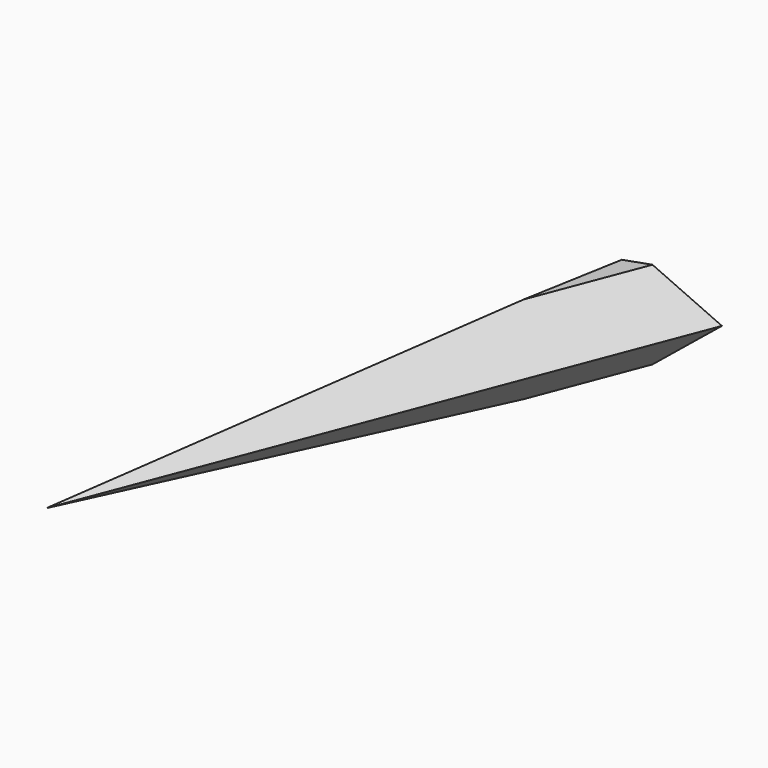
from build123d import *

# Parameters (mm, degrees)
F1_DEPTH = 10
F2_SIZE  = 4.99999


# Not quite as in the source:
# - a fillet or chamfer is up to 0.001 mm smaller than in the source, because OpenCascade refuses the exact size


with BuildPart() as f1:
    # F0 (on Top) → F1 (new body)
    with BuildSketch(Plane.XY):
        Polygon((-26.4395750973, 41.8424181081), (-40.7729081464, 36.8424181081), (-51.4395743695, -23.1575818919), align=None)
    extrude(amount=F1_DEPTH)

    # F2 (size 5 in the source; OpenCascade refuses exactly that, so slightly less here)
    f2_edges = [f1.edges().sort_by_distance(p)[0] for p in [
        (-46.106241, 6.842418, 10),
        (-38.939575, 9.342418, 10),
        (-46.106241, 6.842418, 0),
        (-38.939575, 9.342418, 0),
    ]]
    chamfer(f2_edges, length=F2_SIZE)


solid = f1.part
